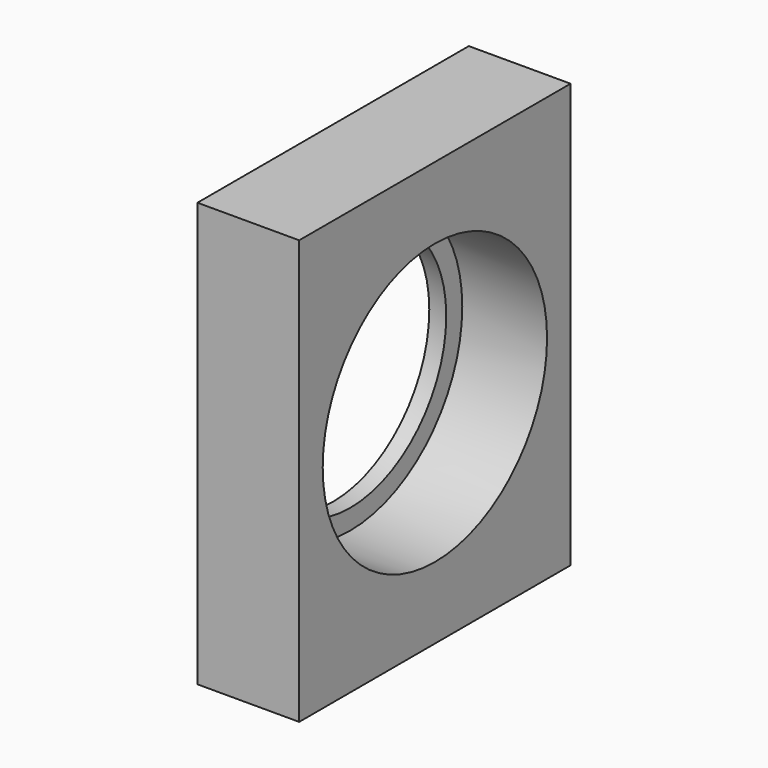
from build123d import *

# Parameters (mm, degrees)
F0_W     = 25.4
F0_H     = 31.75
F0_R     = 10.5
F1_DEPTH = 7.62
F3_D     = 4.7625
F3_DEPTH = 4.7625
F3_TIP   = 1.4307993491
F0_R_2   = 9
F4_DEPTH = 1.27


# Not quite as in the source:
# - a feature names something its author has since deleted; it is built from what else it names


with BuildPart() as f1:
    # F0 (on Right) → F1 (new body)
    with BuildSketch(Plane.YZ):
        Rectangle(F0_W, F0_H)
        Circle(F0_R, mode=Mode.SUBTRACT)
    extrude(amount=F1_DEPTH)

    # F3
    with Locations(Plane(origin=(0, 0, -15.875), x_dir=(1, 0, 0), z_dir=(0, 0, -1))):
        with Locations((3.81, 6.35), (3.81, -6.35)):
            Hole(F3_D / 2, depth=F3_DEPTH)
            with Locations((0, 0, -(F3_DEPTH + F3_TIP / 2))):  # 118° drill point
                Cone(0, F3_D / 2, F3_TIP, mode=Mode.SUBTRACT)

    # F0 (on Right) → F4 (join)
    with BuildSketch(Plane.YZ):
        Circle(F0_R)
        Circle(F0_R_2, mode=Mode.SUBTRACT)
    extrude(amount=F4_DEPTH)


solid = f1.part
